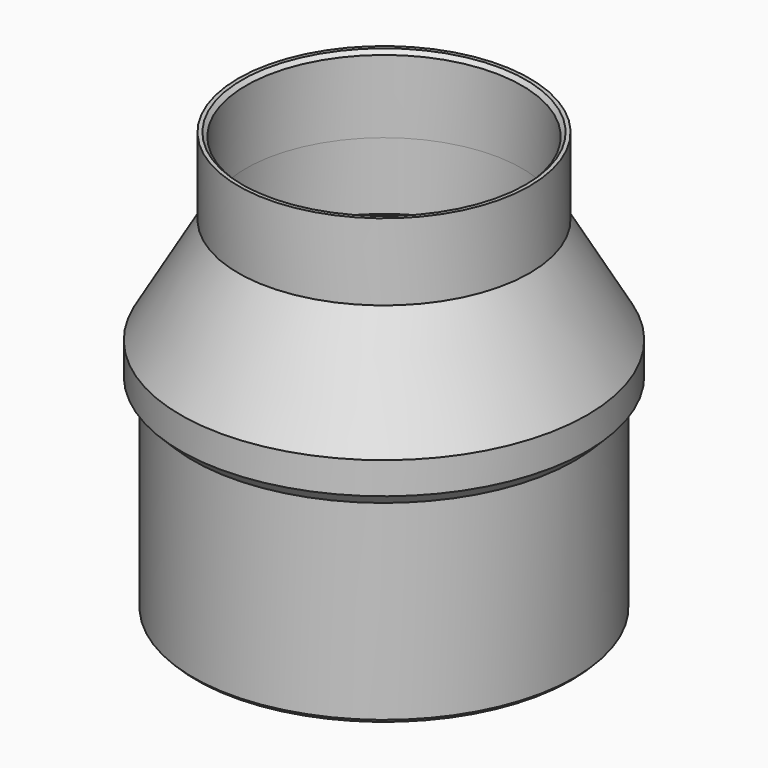
from build123d import *

# Parameters (mm, degrees)
F0_R        = 26.5
F0_R_2      = 24.9
F0_R_3      = 23.5
F0_R_4      = 19
F0_R_5      = 18
F1_DEPTH    = 20
F2_DEPTH    = 25
F3_START    = 20
F3_DEPTH    = 10
F4_SIZE2    = 13.8564064606
F4_SIZE     = 8
F5_SIZE     = 0.5
F6_SIZE     = 0.5
F7_S5_R     = 24.9
F7_T6_DEPTH = 39
F8_S5_R     = 23.5
F8_T6_DEPTH = 37


# Not quite as in the source:
# - a fillet or chamfer that OpenCascade refuses, or shapes differently, is made with other operations: its cross-section is extruded or revolved along the edge and cut away or added


with BuildPart() as f1:
    # F0 (on Top) → F1 (new body)
    with BuildSketch(Plane.XY):
        Circle(F0_R)
        Circle(F0_R_2, mode=Mode.SUBTRACT)
        Circle(F0_R_2)
        Circle(F0_R_3, mode=Mode.SUBTRACT)
        Circle(F0_R_3)
        Circle(F0_R_4, mode=Mode.SUBTRACT)
        Circle(F0_R_4)
        Circle(F0_R_5, mode=Mode.SUBTRACT)
    extrude(amount=F1_DEPTH)

    # F0 (on Top) → F2 (join)
    with BuildSketch(Plane.XY):
        Circle(F0_R_2)
        Circle(F0_R_3, mode=Mode.SUBTRACT)
    extrude(amount=-F2_DEPTH)

    # F4
    f4_edges = [f1.edges().sort_by_distance(p)[0] for p in [
        (-26.5, 0, 20),
    ]]
    f4_side = f1.faces().sort_by_distance((-25.750467, 0, 20))[0]
    chamfer(f4_edges, length=F4_SIZE, length2=F4_SIZE2, reference=f4_side)

    # F6
    f6_edges = [f1.edges().sort_by_distance(p)[0] for p in [
        (-24.9, 0, -25),
    ]]
    chamfer(f6_edges, length=F6_SIZE)

    # F7: chamfer of 2 on 1 edges, made by hand


with BuildPart() as f3:
    # F0 (on Top) → F3 (new body)
    with BuildSketch(Plane.XY.offset(F3_START)):
        Circle(F0_R_4)
        Circle(F0_R_5, mode=Mode.SUBTRACT)
    extrude(amount=F3_DEPTH)

    # F5
    f5_edges = [f3.edges().sort_by_distance(p)[0] for p in [
        (-18, 0, 30),
    ]]
    chamfer(f5_edges, length=F5_SIZE)


with BuildPart() as f7_tool2:
    # F7_s3 → F7_t4 (revolve)
    with BuildSketch(Plane.XZ):
        Polygon((24.5, 0), (26.5, 2), (26.5, 0), align=None)
    revolve(axis=Axis((0, 0, 0), (0, 0, 1)))

    # F7_s5 → F7_t6 (cut, symmetric)
    with BuildSketch(Plane.XY.offset(1)):
        Circle(F7_S5_R)
    extrude(amount=F7_T6_DEPTH, both=True, mode=Mode.SUBTRACT)


with BuildPart() as f1_1:
    add(f1.part)

    # F7_t1: cut F7_tool2
    add(f7_tool2.part, mode=Mode.SUBTRACT)

    # F8: chamfer of 6.5 x 11.2583302492 on 1 edges, made by hand


with BuildPart() as f8_tool2:
    # F8_s3 → F8_t4 (revolve)
    with BuildSketch(Plane.XZ):
        Polygon((18, 11.2583302492), (24.5, 0), (18, 0), align=None)
    revolve(axis=Axis((0, 0, 0), (0, 0, 1)))

    # F8_s5 → F8_t6 (intersect, symmetric)
    with BuildSketch(Plane.XY.offset(5.6)):
        Circle(F8_S5_R)
    extrude(amount=F8_T6_DEPTH, both=True, mode=Mode.INTERSECT)


with BuildPart() as f1_2:
    add(f1_1.part)

    # F8_t1: cut F8_tool2
    add(f8_tool2.part, mode=Mode.SUBTRACT)


solid = Compound([f3.part, f1_2.part])
